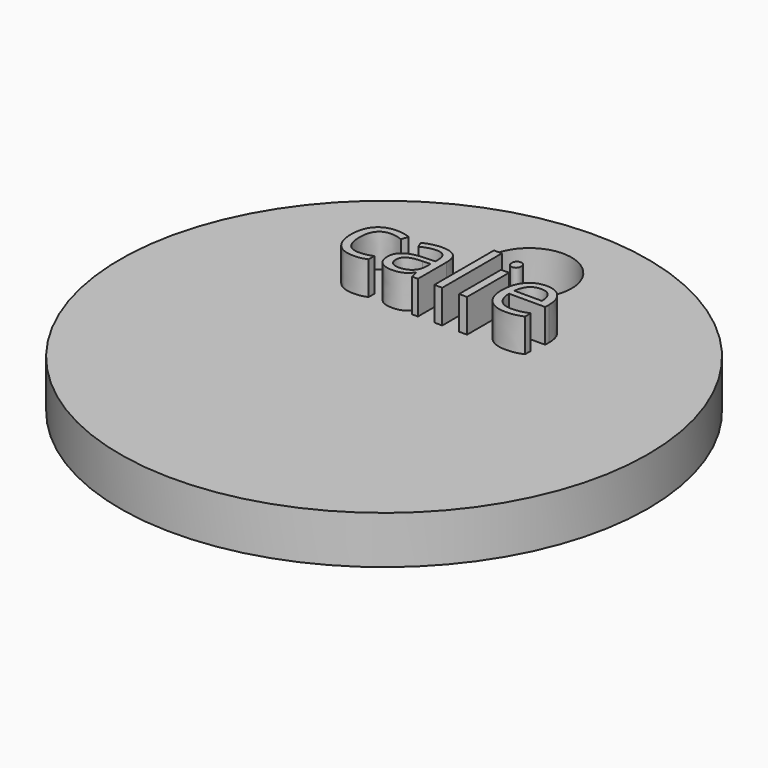
from build123d import *

# Parameters (mm, degrees)
F0_R         = 55.2502178018
F1_DEPTH     = 10
F2_R         = 8.8244820929
F3_DEPTH     = 25
F4_TEXT_SIZE = 20.5255084427
F5_DEPTH     = 6.9550108165


# Not quite as in the source:
# - Text() gives the source's letters only with a copy of the font that has no kerning and outlines rounded to 1/6400 em; it was checked with that copy


with BuildPart() as f1:
    # F0 (on Top) → F1 (new body)
    with BuildSketch(Plane.XY):
        Circle(F0_R)
    extrude(amount=F1_DEPTH)

    # F2 (on face) → F3 (cut)
    with BuildSketch(Plane.XY.offset(10)):
        with Locations((0, 38.0104333162)):
            Circle(F2_R)
    extrude(amount=-F3_DEPTH, mode=Mode.SUBTRACT)

    # F4 (on face) → F5 (join)
    with BuildSketch(Plane.XY.offset(10)):
        with Locations((-24.1154916584, 14.5929756117)):
            Text('calie', F4_TEXT_SIZE, font='Open Sans', text_align=(TextAlign.LEFT, TextAlign.BOTTOM))
    extrude(amount=F5_DEPTH)


solid = f1.part
